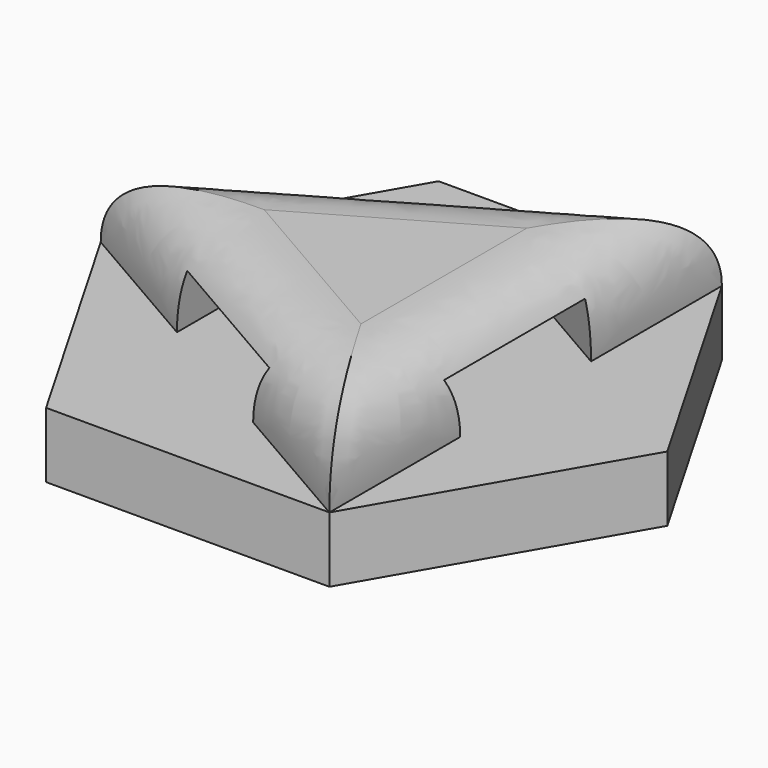
from build123d import *

# Parameters (mm, degrees)
F1_DEPTH    = 4
F3_DEPTH    = 5
F5_DEPTH    = 3
F6_T1_DEPTH = 55
F6_T3_DEPTH = 55
F6_T5_DEPTH = 55


# Not quite as in the source:
# - a fillet or chamfer that OpenCascade refuses, or shapes differently, is made with other operations: its cross-section is extruded or revolved along the edge and cut away or added


with BuildPart() as f1:
    # F0 (on Top) → F1 (new body)
    with BuildSketch(Plane.XY):
        Polygon((17.3205080757, 0), (8.6602540378, 15), (-8.6602540378, 15), (-17.3205080757, 0), (-8.6602540378, -15), (8.6602540378, -15), align=None)
    extrude(amount=F1_DEPTH)

    # F2 (on face) → F3 (join)
    with BuildSketch(Plane.XY.offset(4)):
        Polygon((8.6602540378, -15), (8.6602540378, 15), (-17.3205080757, 0), align=None)
    extrude(amount=F3_DEPTH)

    # F4 (on face) → F5 (cut)
    with BuildSketch(Plane.XY.offset(4)):
        Polygon((8.6602540378, -5), (8.6602540378, 5), (0, 10), (-8.6602540378, 5), (-8.6602540378, -5), (0, -10), align=None)
    extrude(amount=F5_DEPTH, mode=Mode.SUBTRACT)

    # F6: fillet of radius 5 on 3 edges, made by hand

    # F6_s2 → F6_t1 (cut)
    with BuildSketch(Plane(origin=(-23.8156986041, 13.75, 0), x_dir=(0, 0, 1), z_dir=(0.8660254038, -0.5, 0))):
        with BuildLine():
            add(Edge.make_bspline(
                [(4, 8.6602540378), (9, 8.6602540378), (9, 3.6602540378)],
                knots=[0, 0, 0, 1, 1, 1], degree=2, weights=[1, 1, 1]))
            Line((9, 3.6602540378), (9, 8.6602540378))
            Line((9, 8.6602540378), (4, 8.6602540378))
        make_face()
    extrude(amount=F6_T1_DEPTH, mode=Mode.SUBTRACT)

    # F6_s4 → F6_t3 (cut)
    with BuildSketch(Plane.XZ.offset(-27.5)):
        with BuildLine():
            add(Edge.make_bspline(
                [(8.6602540378, 4), (8.6602540378, 9), (3.6602540378, 9)],
                knots=[0, 0, 0, 1, 1, 1], degree=2, weights=[1, 1, 1]))
            Line((3.6602540378, 9), (8.6602540378, 9))
            Line((8.6602540378, 9), (8.6602540378, 4))
        make_face()
    extrude(amount=F6_T3_DEPTH, mode=Mode.SUBTRACT)

    # F6_s6 → F6_t5 (cut)
    with BuildSketch(Plane(origin=(23.8156986041, 13.75, 0), x_dir=(0, 0, 1), z_dir=(-0.8660254038, -0.5, 0))):
        with BuildLine():
            add(Edge.make_bspline(
                [(4, 8.6602540378), (9, 8.6602540378), (9, 3.6602540378)],
                knots=[0, 0, 0, 1, 1, 1], degree=2, weights=[1, 1, 1]))
            Line((9, 3.6602540378), (9, 8.6602540378))
            Line((9, 8.6602540378), (4, 8.6602540378))
        make_face()
    extrude(amount=F6_T5_DEPTH, mode=Mode.SUBTRACT)


solid = f1.part
